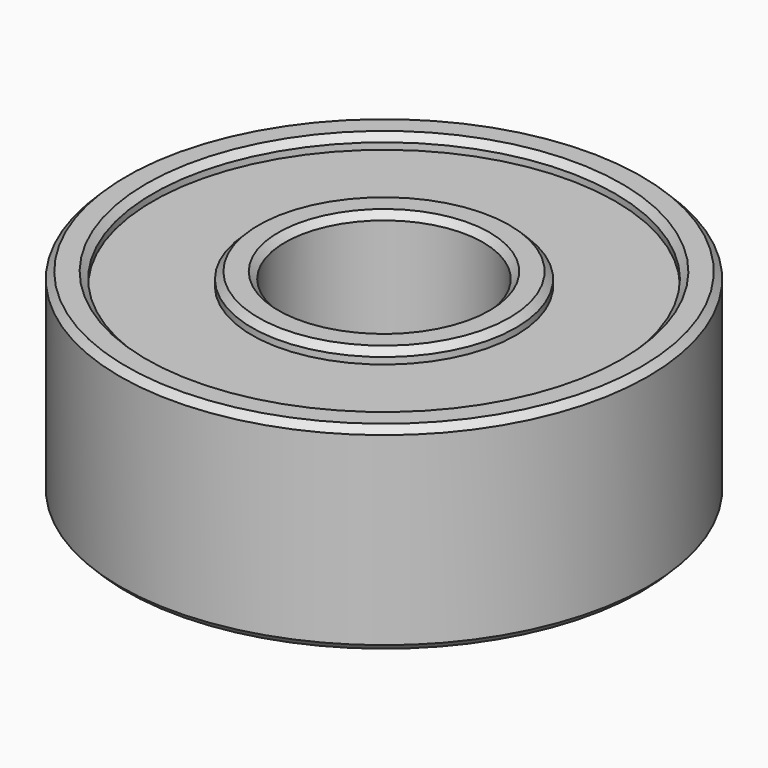
from build123d import *

# Parameters (mm, degrees)
F0_R      = 2
F0_R_2    = 1.5
F1_DEPTH  = 3
F0_R_3    = 4
F0_R_4    = 3.5
F2_START  = 0.2
F2_DEPTH  = 2.6
F3_SIZE   = 0.1
F3_2_SIZE = 0.1


with BuildPart() as f1:
    # F0 (on Top) → F1 (new body)
    with BuildSketch(Plane.XY):
        Circle(F0_R)
        Circle(F0_R_2, mode=Mode.SUBTRACT)
    extrude(amount=F1_DEPTH)

    # F3
    f3_edges = [f1.edges().sort_by_distance(p)[0] for p in [
        (-2, 0, 0),
        (-1.5, 0, 0),
        (-2, 0, 3),
        (-1.5, 0, 3),
    ]]
    chamfer(f3_edges, length=F3_SIZE)


with BuildPart() as f1b:
    # F0 (on Top) → F1, piece 2 (new body)
    with BuildSketch(Plane.XY):
        Circle(F0_R_3)
        Circle(F0_R_4, mode=Mode.SUBTRACT)
    extrude(amount=F1_DEPTH)

    # F3#2
    f3_2_edges = [f1b.edges().sort_by_distance(p)[0] for p in [
        (-4, 0, 3),
        (-3.5, 0, 3),
        (-4, 0, 0),
        (-3.5, 0, 0),
    ]]
    chamfer(f3_2_edges, length=F3_2_SIZE)


with BuildPart() as f2:
    # F0 (on Top) → F2 (new body)
    with BuildSketch(Plane.XY.offset(F2_START)):
        Circle(F0_R_4)
        Circle(F0_R, mode=Mode.SUBTRACT)
    extrude(amount=F2_DEPTH)


solid = Compound([f1.part, f1b.part, f2.part])
